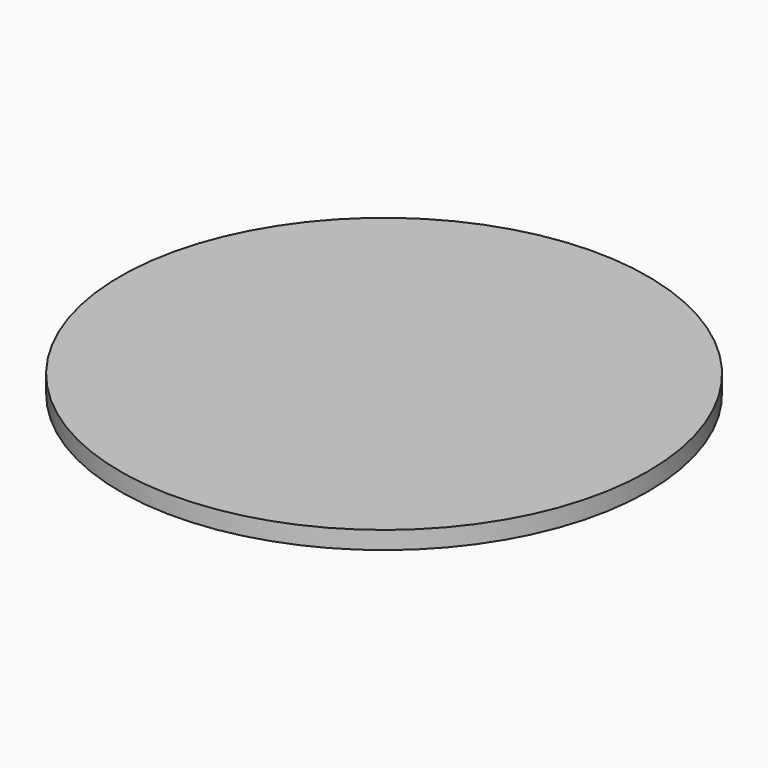
from build123d import *

# Parameters (mm, degrees)
F0_R     = 148.5
F1_DEPTH = 10
F2_R     = 146.5
F2_R_2   = 142
F3_DEPTH = 5


# Not quite as in the source:
# - a feature names something its author has since deleted; it is built from what else it names


with BuildPart() as f1:
    # F0 (on Top) → F1 (new body)
    with BuildSketch(Plane.XY):
        Circle(F0_R)
    extrude(amount=F1_DEPTH)

    # F2 (on face) → F3 (cut)
    with BuildSketch(Plane.XY):
        Circle(F2_R)
        Circle(F2_R_2, mode=Mode.SUBTRACT)
    extrude(amount=F3_DEPTH, mode=Mode.SUBTRACT)


solid = f1.part
